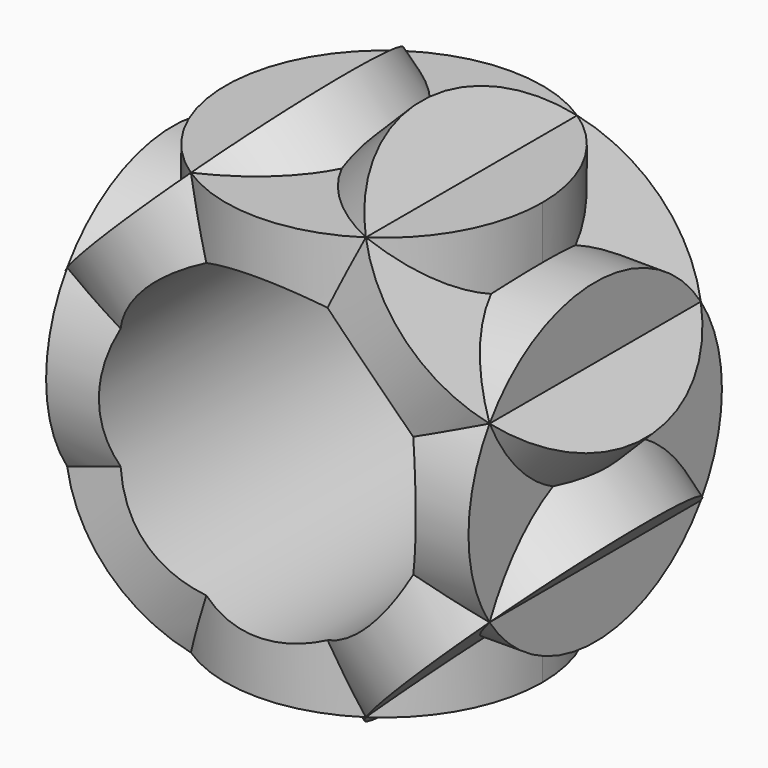
from build123d import *
from build123d import SkipClean  # not in build123d's __all__

# Parameters (mm, degrees)
F0_R      = 19.05
F1_DEPTH  = 25.4
F2_R      = 19.05
F3_DEPTH  = 25.4
F4_R      = 19.05
F5_DEPTH  = 25.4
F7_R      = 19.05
F8_DEPTH  = 25.4
F10_R     = 19.05
F11_DEPTH = 25.4
F12_R     = 19.05
F13_DEPTH = 50.8


# Not quite as in the source:
# - a pattern or mirror of a feature is missing from the dataset's text; its kind, count and spacing are read off the source's solid


with BuildPart() as f1:
    # F0 (on Right) → F1 (new body, symmetric)
    with BuildSketch(Plane.YZ):
        Circle(F0_R)
    extrude(amount=F1_DEPTH, both=True)

    # F1_copies: F1 across plane


with BuildPart() as f1_1:
    add(f1.part, clean=False)
    add(f1.part.mirror(Plane(origin=(0, 0, 0), x_dir=(-0.9238795325, 0, -0.3826834323), z_dir=(0.3826834323, 0, -0.9238795325))), clean=False)

    # F2 (on Top) → F3 (join, symmetric)
    with BuildSketch(Plane.XY):
        Circle(F2_R)
    with SkipClean():  # cleaning this boolean's faces spoils the solid; the shape is the same uncleaned
        extrude(amount=F3_DEPTH, both=True)

    # F4 (on Front) → F5 (join, symmetric)
    with BuildSketch(Plane.XZ):
        Circle(F4_R)
    with SkipClean():  # cleaning this boolean's faces spoils the solid; the shape is the same uncleaned
        extrude(amount=F5_DEPTH, both=True)

    # F7 (on face) → F8 (join, symmetric)
    with BuildSketch(Plane(origin=(0, 0, 0), x_dir=(0, 1, 0), z_dir=(0.7071067812, 0, -0.7071067812))):
        Circle(F7_R)
    with SkipClean():  # cleaning this boolean's faces spoils the solid; the shape is the same uncleaned
        extrude(amount=F8_DEPTH, both=True)

    # F10 (on face) → F11 (join, symmetric)
    with BuildSketch(Plane(origin=(0, 0, 0), x_dir=(0, 1, 0), z_dir=(0.7071067812, 0, 0.7071067812))):
        Circle(F10_R)
    with SkipClean():  # cleaning this boolean's faces spoils the solid; the shape is the same uncleaned
        extrude(amount=F11_DEPTH, both=True)

    # F12 (on face) → F13 (cut)
    with BuildSketch(Plane(origin=(0, 25.4, 0), x_dir=(-1, 0, 0), z_dir=(0, 1, 0))):
        Circle(F12_R)
    with SkipClean():  # cleaning this boolean's faces spoils the solid; the shape is the same uncleaned
        extrude(amount=-F13_DEPTH, mode=Mode.SUBTRACT)


solid = f1_1.part
